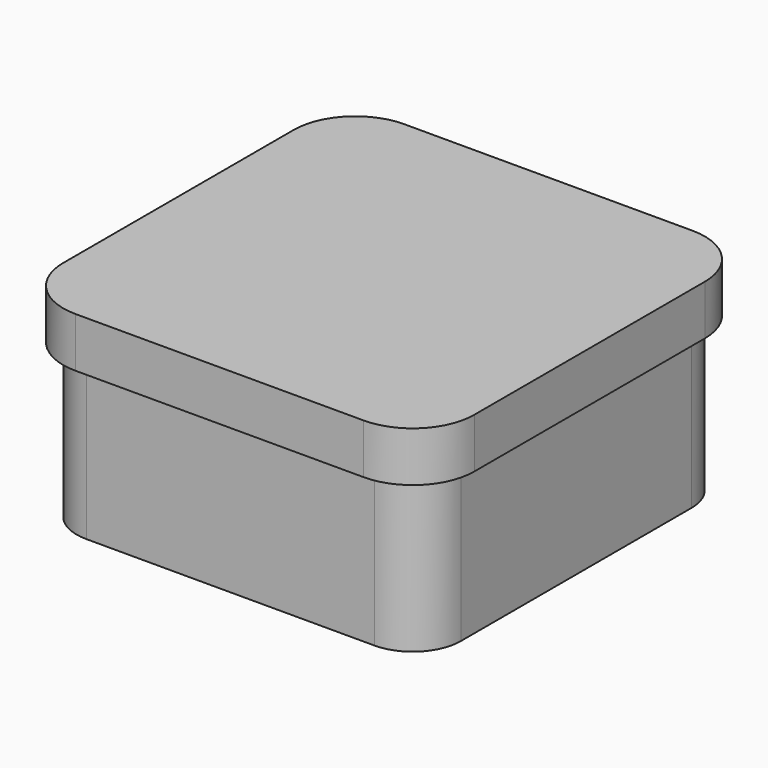
from build123d import *

# Parameters (mm, degrees)
F0_W            = 40
F0_H            = 40
F1_DEPTH        = 20
F2_R            = 5
F3_T            = -1.2
F5_DEPTH        = 1.2
F6_DEPTH        = 4
F8_DEPTH        = 1.7
F8_COPIES_COUNT = 4
F9_DEPTH        = 1.5
F9_COPIES_COUNT = 4


# Not quite as in the source:
# - a pattern or mirror of a feature is missing from the dataset's text; its kind, count and spacing are read off the source's solid


with BuildPart() as f1:
    # F0 (on Top) → F1 (new body)
    with BuildSketch(Plane.XY):
        Rectangle(F0_W, F0_H)
    extrude(amount=F1_DEPTH)

    # F2
    f2_edges = [f1.edges().sort_by_distance(p)[0] for p in [
        (20, -20, 10),
        (20, 20, 10),
        (-20, -20, 10),
        (-20, 20, 10),
    ]]
    fillet(f2_edges, radius=F2_R)

    # F3
    f3_openings = [f1.faces().sort_by_distance(p)[0] for p in [
        (0, 0, 20),
    ]]
    offset(amount=F3_T, openings=f3_openings)

    # F7 (on Front) → F8 (cut, symmetric)
    with BuildSketch(Plane.XZ):
        with BuildLine():
            Line((19.4470588235, 17.9117647059), (20.2, 16.5))
            Line((20.2, 16.5), (20.2, 18.5))
            Line((20.2, 18.5), (19.8, 18.5))
            ThreePointArc((19.8, 18.5), (19.4570028297, 18.3057983022), (19.4470588235, 17.9117647059))
        make_face()
        with BuildLine():
            Line((19.8, 18.5), (20.2, 18.5))
            Line((20.2, 18.5), (20.2, 18.9))
            ThreePointArc((20.2, 18.9), (20.0828427125, 18.6171572875), (19.8, 18.5))
        make_face()
        with BuildLine():
            Line((20.2, 16.0750016282), (20.2, 16.5))
            Line((20.2, 16.5), (19.4470588235, 17.9117647059))
            ThreePointArc((19.4470588235, 17.9117647059), (19.4570028297, 18.3057983022), (19.8, 18.5))
            ThreePointArc((19.8, 18.5), (20.0828427125, 18.6171572875), (20.2, 18.9))
            Line((20.2, 18.9), (20.2, 19.45))
            Line((20.2, 19.45), (19.9891899905, 18.8351351096))
            ThreePointArc((19.9891899905, 18.8351351096), (19.91624818, 18.7372527508), (19.8, 18.6999992338))
            ThreePointArc((19.8, 18.6999992338), (19.2855049016, 18.408697059), (19.2705889114, 17.8176474194))
            Line((19.2705889114, 17.8176474194), (20.2, 16.0750016282))
        make_face()
    f8 = extrude(amount=F8_DEPTH, both=True, mode=Mode.SUBTRACT)

    # F8_copies: F8 ×4 about axis
    f8_copies_axis = Axis((0, 0, 0), (0, 0, 1))
    for i in range(1, F8_COPIES_COUNT):
        add(f8.rotate(f8_copies_axis, i * 360 / F8_COPIES_COUNT), mode=Mode.SUBTRACT)


with BuildPart() as f5:
    # F4 (on face) → F5 (new body)
    with BuildSketch(Plane.XY.offset(20)):
        with BuildLine():
            Line((-21.4, 15), (-21.4, -15))
            ThreePointArc((-21.4, -15), (-19.5254833996, -19.5254833996), (-15, -21.4))
            Line((-15, -21.4), (15, -21.4))
            ThreePointArc((15, -21.4), (19.5254833996, -19.5254833996), (21.4, -15))
            Line((21.4, -15), (21.4, 15))
            ThreePointArc((21.4, 15), (19.5254833996, 19.5254833996), (15, 21.4))
            Line((15, 21.4), (-15, 21.4))
            ThreePointArc((-15, 21.4), (-19.5254833996, 19.5254833996), (-21.4, 15))
        make_face()
        with BuildLine():
            ThreePointArc((-15, -20.2), (-18.6769552622, -18.6769552622), (-20.2, -15))
            Line((-20.2, -15), (-20.2, 15))
            ThreePointArc((-20.2, 15), (-18.6769552622, 18.6769552622), (-15, 20.2))
            Line((-15, 20.2), (15, 20.2))
            ThreePointArc((15, 20.2), (18.6769552622, 18.6769552622), (20.2, 15))
            Line((20.2, 15), (20.2, -15))
            ThreePointArc((20.2, -15), (18.6769552622, -18.6769552622), (15, -20.2))
            Line((15, -20.2), (-15, -20.2))
        make_face(mode=Mode.SUBTRACT)
        with BuildLine():
            Line((-20.2, 15), (-20.2, -15))
            ThreePointArc((-20.2, -15), (-18.6769552622, -18.6769552622), (-15, -20.2))
            Line((-15, -20.2), (15, -20.2))
            ThreePointArc((15, -20.2), (18.6769552622, -18.6769552622), (20.2, -15))
            Line((20.2, -15), (20.2, 15))
            ThreePointArc((20.2, 15), (18.6769552622, 18.6769552622), (15, 20.2))
            Line((15, 20.2), (-15, 20.2))
            ThreePointArc((-15, 20.2), (-18.6769552622, 18.6769552622), (-20.2, 15))
        make_face()
        with BuildLine():
            Line((15, -20), (-15, -20))
            ThreePointArc((-15, -20), (-18.5355339059, -18.5355339059), (-20, -15))
            Line((-20, -15), (-20, 15))
            ThreePointArc((-20, 15), (-18.5355339059, 18.5355339059), (-15, 20))
            Line((-15, 20), (15, 20))
            ThreePointArc((15, 20), (18.5355339059, 18.5355339059), (20, 15))
            Line((20, 15), (20, -15))
            ThreePointArc((20, -15), (18.5355339059, -18.5355339059), (15, -20))
        make_face(mode=Mode.SUBTRACT)
        with BuildLine():
            ThreePointArc((-20, -15), (-18.5355339059, -18.5355339059), (-15, -20))
            Line((-15, -20), (15, -20))
            ThreePointArc((15, -20), (18.5355339059, -18.5355339059), (20, -15))
            Line((20, -15), (20, 15))
            ThreePointArc((20, 15), (18.5355339059, 18.5355339059), (15, 20))
            Line((15, 20), (-15, 20))
            ThreePointArc((-15, 20), (-18.5355339059, 18.5355339059), (-20, 15))
            Line((-20, 15), (-20, -15))
        make_face()
        with BuildLine():
            ThreePointArc((-18.8, 15), (-17.6870057685, 17.6870057685), (-15, 18.8))
            Line((-15, 18.8), (15, 18.8))
            ThreePointArc((15, 18.8), (17.6870057685, 17.6870057685), (18.8, 15))
            Line((18.8, 15), (18.8, -15))
            ThreePointArc((18.8, -15), (17.6870057685, -17.6870057685), (15, -18.8))
            Line((15, -18.8), (-15, -18.8))
            ThreePointArc((-15, -18.8), (-17.6870057685, -17.6870057685), (-18.8, -15))
            Line((-18.8, -15), (-18.8, 15))
        make_face(mode=Mode.SUBTRACT)
        with BuildLine():
            Line((15, 18.8), (-15, 18.8))
            ThreePointArc((-15, 18.8), (-17.6870057685, 17.6870057685), (-18.8, 15))
            Line((-18.8, 15), (-18.8, -15))
            ThreePointArc((-18.8, -15), (-17.6870057685, -17.6870057685), (-15, -18.8))
            Line((-15, -18.8), (15, -18.8))
            ThreePointArc((15, -18.8), (17.6870057685, -17.6870057685), (18.8, -15))
            Line((18.8, -15), (18.8, 15))
            ThreePointArc((18.8, 15), (17.6870057685, 17.6870057685), (15, 18.8))
        make_face()
    extrude(amount=F5_DEPTH)

    # F4 (on face) → F6 (join)
    with BuildSketch(Plane.XY.offset(20)):
        with BuildLine():
            Line((-21.4, 15), (-21.4, -15))
            ThreePointArc((-21.4, -15), (-19.5254833996, -19.5254833996), (-15, -21.4))
            Line((-15, -21.4), (15, -21.4))
            ThreePointArc((15, -21.4), (19.5254833996, -19.5254833996), (21.4, -15))
            Line((21.4, -15), (21.4, 15))
            ThreePointArc((21.4, 15), (19.5254833996, 19.5254833996), (15, 21.4))
            Line((15, 21.4), (-15, 21.4))
            ThreePointArc((-15, 21.4), (-19.5254833996, 19.5254833996), (-21.4, 15))
        make_face()
        with BuildLine():
            ThreePointArc((-15, -20.2), (-18.6769552622, -18.6769552622), (-20.2, -15))
            Line((-20.2, -15), (-20.2, 15))
            ThreePointArc((-20.2, 15), (-18.6769552622, 18.6769552622), (-15, 20.2))
            Line((-15, 20.2), (15, 20.2))
            ThreePointArc((15, 20.2), (18.6769552622, 18.6769552622), (20.2, 15))
            Line((20.2, 15), (20.2, -15))
            ThreePointArc((20.2, -15), (18.6769552622, -18.6769552622), (15, -20.2))
            Line((15, -20.2), (-15, -20.2))
        make_face(mode=Mode.SUBTRACT)
    extrude(amount=-F6_DEPTH)

    # F7 (on Front) → F9 (join, symmetric)
    with BuildSketch(Plane.XZ):
        with BuildLine():
            Line((19.4470588235, 17.9117647059), (20.2, 16.5))
            Line((20.2, 16.5), (20.2, 18.5))
            Line((20.2, 18.5), (19.8, 18.5))
            ThreePointArc((19.8, 18.5), (19.4570028297, 18.3057983022), (19.4470588235, 17.9117647059))
        make_face()
    f9 = extrude(amount=F9_DEPTH, both=True)

    # F9_copies: F9 ×4 about axis
    f9_copies_axis = Axis((0, 0, 0), (0, 0, 1))
    for i in range(1, F9_COPIES_COUNT):
        add(f9.rotate(f9_copies_axis, i * 360 / F9_COPIES_COUNT))


solid = Compound([f1.part, f5.part])
